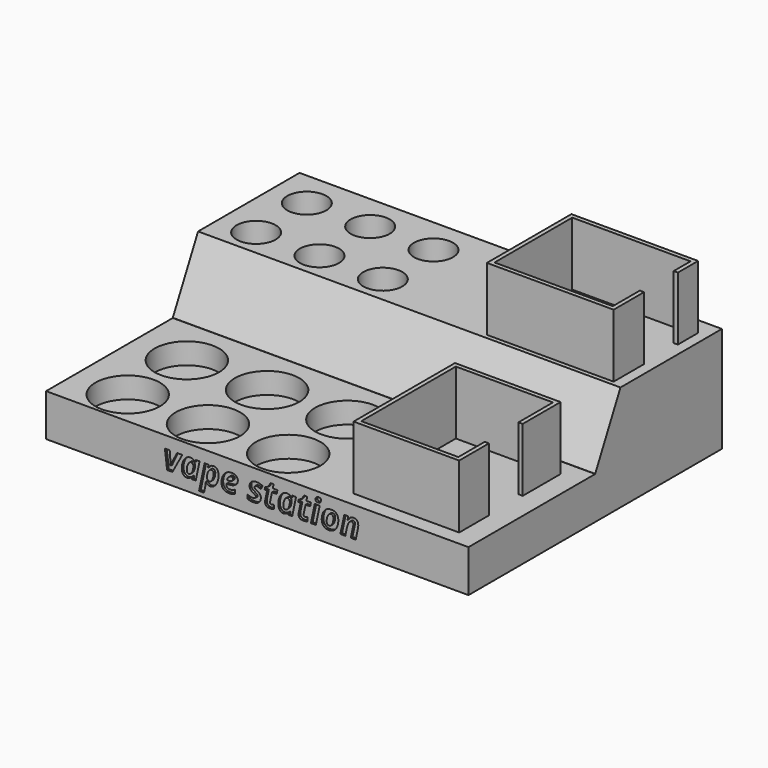
from build123d import *

# Parameters (mm, degrees)
F0_W          = 200
F0_H          = 150
F1_DEPTH      = 20
F2_R          = 15.25
F2_R_2        = 4
F3_DEPTH      = 10
F4_DEPTH      = 18
F2_W          = 50
F2_H          = 60
F5_DEPTH      = 30
F6_W          = 20
F6_H          = 30
F7_DEPTH      = 2.5
F9_DEPTH      = 30
F2_W_2        = 200
F2_H_2        = 75
F10_DEPTH     = 30
F11_R         = 9.25
F12_DEPTH     = 30
F13_DEPTH     = 30
F14_TEXT_SIZE = 15.8084039059
F15_DEPTH     = 1
F17_DEPTH     = 200


# Not quite as in the source:
# - Text() gives the source's letters only with a copy of the font that has no kerning and outlines rounded to 1/6400 em; it was checked with that copy


with BuildPart() as f1:
    # F0 (on Top) → F1 (new body)
    with BuildSketch(Plane.XY):
        Rectangle(F0_W, F0_H)
    extrude(amount=F1_DEPTH)

    # F2 (on face) → F3 (cut)
    with BuildSketch(Plane.XY.offset(20)):
        with Locations((-74.75, -23.25)):
            Circle(F2_R)
        with Locations((-74.75, -23.25)):
            Circle(F2_R_2, mode=Mode.SUBTRACT)
        with Locations((-36.75, -23.25)):
            Circle(F2_R)
        with Locations((-36.75, -23.25)):
            Circle(F2_R_2, mode=Mode.SUBTRACT)
        with Locations((1.25, -23.25)):
            Circle(F2_R)
        with Locations((1.25, -23.25)):
            Circle(F2_R_2, mode=Mode.SUBTRACT)
        with Locations((1.25, -58.25)):
            Circle(F2_R)
        with Locations((1.25, -58.25)):
            Circle(F2_R_2, mode=Mode.SUBTRACT)
        with Locations((-36.75, -58.25)):
            Circle(F2_R)
        with Locations((-36.75, -58.25)):
            Circle(F2_R_2, mode=Mode.SUBTRACT)
        with Locations((-74.75, -58.25)):
            Circle(F2_R)
        with Locations((-74.75, -58.25)):
            Circle(F2_R_2, mode=Mode.SUBTRACT)
    extrude(amount=-F3_DEPTH, mode=Mode.SUBTRACT)

    # F4 (cut): faces of the model
    f4_faces = [f1.faces().sort_by_distance(p)[0] for p in [
        (-74.75, -23.25, 20),
        (-36.75, -23.25, 20),
        (1.25, -23.25, 20),
        (1.25, -58.25, 20),
        (-36.75, -58.25, 20),
        (-74.75, -58.25, 20),
    ]]
    extrude(f4_faces, amount=-F4_DEPTH, mode=Mode.SUBTRACT)

    # F2 (on face) → F5 (join)
    with BuildSketch(Plane.XY.offset(20)):
        with Locations((65, -38)):
            Rectangle(F2_W, F2_H)
    extrude(amount=F5_DEPTH)

    # F6 (on face) → F7 (cut)
    with BuildSketch(Plane.YZ.offset(90)):
        with Locations((-40.3822565079, 35)):
            Rectangle(F6_W, F6_H)
    extrude(amount=-F7_DEPTH, mode=Mode.SUBTRACT)

    # F8 (on face) → F9 (cut, through all)
    with BuildSketch(Plane.XY.offset(50)):
        Polygon((88, -30.3822565079), (88, -10), (42, -10), (42, -66), (88, -66), (88, -50.3822565079), (87.5, -50.3822565079), (87.5, -30.3822565079), align=None)
    extrude(amount=-F9_DEPTH, mode=Mode.SUBTRACT)

    # F2 (on face) → F10 (join)
    with BuildSketch(Plane.XY.offset(20)):
        with Locations((0, 37.5)):
            Rectangle(F2_W_2, F2_H_2)
    extrude(amount=F10_DEPTH)

    # F11 (on face) → F12 (cut)
    with BuildSketch(Plane.XY.offset(50)):
        with Locations((-82.75, 57.75)):
            Circle(F11_R)
        with Locations((-52.75, 57.75)):
            Circle(F11_R)
        with Locations((-52.75, 27.75)):
            Circle(F11_R)
        with Locations((-82.75, 27.75)):
            Circle(F11_R)
        with Locations((-22.75, 27.75)):
            Circle(F11_R)
        with Locations((-22.75, 57.75)):
            Circle(F11_R)
    extrude(amount=-F12_DEPTH, mode=Mode.SUBTRACT)

    # F11 (on face) → F13 (join)
    with BuildSketch(Plane.XY.offset(50)):
        Polygon((95.1280617714, 67), (35.1280617714, 67), (35.1280617714, 17), (95.1280617714, 17), (95.1280617714, 35), (93.1280617714, 35), (93.1280617714, 19), (37.1280617714, 19), (37.1280617714, 65), (93.1280617714, 65), (93.1280617714, 55), (95.1280617714, 55), align=None)
    extrude(amount=F13_DEPTH)

    # F14 (on face) → F15 (cut)
    with BuildSketch(Plane.XZ.offset(75)):
        with Locations((-44.530492276, 5.7498775423)):
            Text('vape station', F14_TEXT_SIZE, font='Open Sans', font_style=FontStyle.BOLDITALIC, text_align=(TextAlign.LEFT, TextAlign.BOTTOM))
    extrude(amount=-F15_DEPTH, mode=Mode.SUBTRACT)

    # F16 (on face) → F17 (cut, through all)
    with BuildSketch(Plane(origin=(-100, 0, 0), x_dir=(0, -1, 0), z_dir=(-1, 0, 0))):
        Polygon((0, 50), (-14.9592012167, 50), (0, 20.0815975666), align=None)
    extrude(amount=-F17_DEPTH, mode=Mode.SUBTRACT)


solid = f1.part
